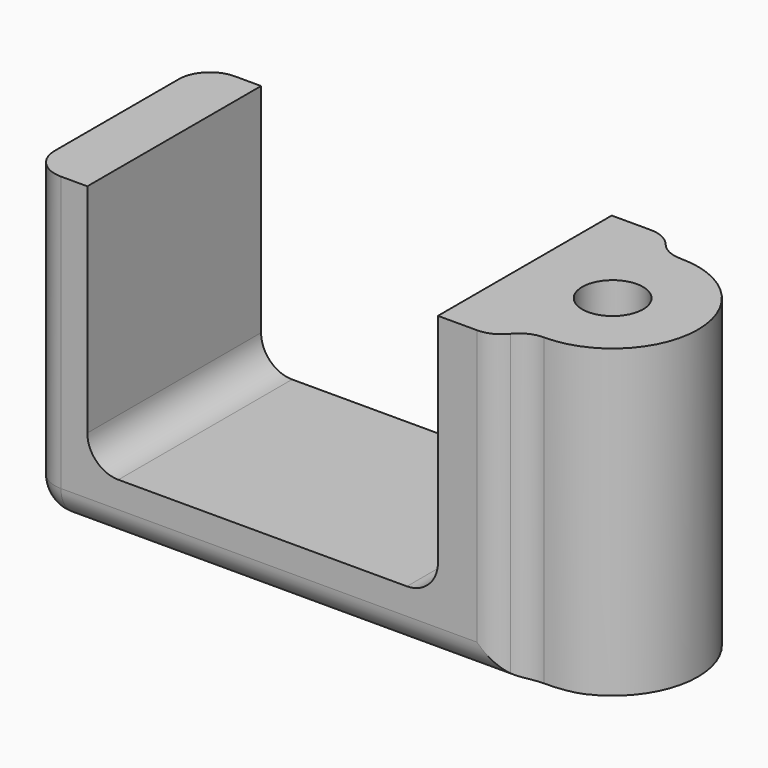
from build123d import *

# Parameters (mm, degrees)
F0_W         = 1.85
F0_H         = 7
F0_W_2       = 11.3
F1_DEPTH     = 1.85
F2_DEPTH     = 8
F3_T1_DEPTH  = 9.85
F3_T3_DEPTH  = 9.85
F3_T5_DEPTH  = 7
F3_T7_DEPTH  = 7
F3_T9_DEPTH  = 12
F4_T1_DEPTH  = 11.35
F4_T3_DEPTH  = 16.5
F4_T5_DEPTH  = 12.8150682373
F4_T8_ANGLE  = 90.0000000053
F4_T10_ANGLE = 90.0000000053


# Not quite as in the source:
# - a fillet or chamfer that OpenCascade refuses, or shapes differently, is made with other operations: its cross-section is extruded or revolved along the edge and cut away or added


with BuildPart() as f1:
    # F0 (on Top) → F1 (new body)
    with BuildSketch(Plane.XY):
        with Locations((-6.575, 0)):
            Rectangle(F0_W, F0_H)
        Rectangle(F0_W_2, F0_H)
        with BuildLine():
            Line((7.5, 0), (7.5, 2.5694551952))
            ThreePointArc((7.5, 2.5694551952), (5.73, 0), (7.5, -2.5694551952))
            Line((7.5, -2.5694551952), (7.5, 0))
        make_face()
        with BuildLine():
            Line((7.5, 2.5694551952), (7.5, 3.5))
            Line((7.5, 3.5), (5.65, 3.5))
            Line((5.65, 3.5), (5.65, -3.5))
            Line((5.65, -3.5), (7.5, -3.5))
            Line((7.5, -3.5), (7.5, -2.5694551952))
            ThreePointArc((7.5, -2.5694551952), (5.73, 0), (7.5, 2.5694551952))
        make_face()
        with BuildLine():
            ThreePointArc((11.23, 0), (10.0400480762, 2.2646743695), (7.5, 2.5694551952))
            Line((7.5, 2.5694551952), (7.5, 0))
            Line((7.5, 0), (7.5, -2.5694551952))
            ThreePointArc((7.5, -2.5694551952), (10.0400480762, -2.2646743695), (11.23, 0))
        make_face()
        with BuildLine():
            ThreePointArc((9.46, 0), (8.48, -0.98), (7.5, 0))
            ThreePointArc((7.5, 0), (8.48, 0.98), (9.46, 0))
        make_face(mode=Mode.SUBTRACT)
    extrude(amount=-F1_DEPTH)

    # F0 (on Top) → F2 (join)
    with BuildSketch(Plane.XY):
        with Locations((-6.575, 0)):
            Rectangle(F0_W, F0_H)
        with BuildLine():
            Line((7.5, 2.5694551952), (7.5, 3.5))
            Line((7.5, 3.5), (5.65, 3.5))
            Line((5.65, 3.5), (5.65, -3.5))
            Line((5.65, -3.5), (7.5, -3.5))
            Line((7.5, -3.5), (7.5, -2.5694551952))
            ThreePointArc((7.5, -2.5694551952), (5.73, 0), (7.5, 2.5694551952))
        make_face()
        with BuildLine():
            Line((7.5, 0), (7.5, 2.5694551952))
            ThreePointArc((7.5, 2.5694551952), (5.73, 0), (7.5, -2.5694551952))
            Line((7.5, -2.5694551952), (7.5, 0))
        make_face()
        with BuildLine():
            ThreePointArc((11.23, 0), (10.0400480762, 2.2646743695), (7.5, 2.5694551952))
            Line((7.5, 2.5694551952), (7.5, 0))
            Line((7.5, 0), (7.5, -2.5694551952))
            ThreePointArc((7.5, -2.5694551952), (10.0400480762, -2.2646743695), (11.23, 0))
        make_face()
        with BuildLine():
            ThreePointArc((9.46, 0), (8.48, -0.98), (7.5, 0))
            ThreePointArc((7.5, 0), (8.48, 0.98), (9.46, 0))
        make_face(mode=Mode.SUBTRACT)
    extrude(amount=F2_DEPTH)

    # F3: fillet of radius 1 on 5 edges, made by hand

    # F3_s2 → F3_t1 (join)
    with BuildSketch(Plane.XY.offset(-1.85)):
        with BuildLine():
            ThreePointArc((7.5, 3.5), (7.8571098794, 2.9584596209), (8.4713837652, 2.7499865019))
            ThreePointArc((8.4713837652, 2.7499865019), (7.9775177584, 2.7037033116), (7.5, 2.5694551952))
            Line((7.5, 2.5694551952), (7.5, 3.5))
        make_face()
    extrude(amount=F3_T1_DEPTH)

    # F3_s4 → F3_t3 (join)
    with BuildSketch(Plane.XY.offset(-1.85)):
        with BuildLine():
            ThreePointArc((7.5, -3.5), (7.8571098794, -2.9584596209), (8.4713837652, -2.7499865019))
            ThreePointArc((8.4713837652, -2.7499865019), (7.9775177584, -2.7037033116), (7.5, -2.5694551952))
            Line((7.5, -2.5694551952), (7.5, -3.5))
        make_face()
    extrude(amount=F3_T3_DEPTH)

    # F3_s6 → F3_t5 (join)
    with BuildSketch(Plane.XZ.offset(-3.5)):
        with BuildLine():
            ThreePointArc((5.65, 1), (5.3571067812, 0.2928932188), (4.65, 0))
            Line((4.65, 0), (5.65, 0))
            Line((5.65, 0), (5.65, 1))
        make_face()
    extrude(amount=F3_T5_DEPTH)

    # F3_s8 → F3_t7 (join)
    with BuildSketch(Plane.XZ.offset(-3.5)):
        with BuildLine():
            ThreePointArc((-4.65, 0), (-5.3571067812, 0.2928932188), (-5.65, 1))
            Line((-5.65, 1), (-5.65, 0))
            Line((-5.65, 0), (-4.65, 0))
        make_face()
    extrude(amount=F3_T7_DEPTH)

    # F3_s10 → F3_t9 (cut)
    with BuildSketch(Plane.XZ.offset(-6)):
        with BuildLine():
            ThreePointArc((-7.5, -0.85), (-7.2071067812, -1.5571067812), (-6.5, -1.85))
            Line((-6.5, -1.85), (-7.5, -1.85))
            Line((-7.5, -1.85), (-7.5, -0.85))
        make_face()
    extrude(amount=F3_T9_DEPTH, mode=Mode.SUBTRACT)

    # F4: fillet of radius 1 on 8 edges, made by hand

    # F4_s2 → F4_t1 (cut)
    with BuildSketch(Plane.XY.offset(-0.85)):
        with BuildLine():
            ThreePointArc((-7.5, 2.5), (-7.2071067812, 3.2071067812), (-6.5, 3.5))
            Line((-6.5, 3.5), (-7.5, 3.5))
            Line((-7.5, 3.5), (-7.5, 2.5))
        make_face()
        with BuildLine():
            ThreePointArc((-7.5, -2.5), (-7.2071067812, -3.2071067812), (-6.5, -3.5))
            Line((-6.5, -3.5), (-7.5, -3.5))
            Line((-7.5, -3.5), (-7.5, -2.5))
        make_face()
    extrude(amount=F4_T1_DEPTH, mode=Mode.SUBTRACT)

    # F4_s4 → F4_t3 (cut)
    with BuildSketch(Plane.YZ.offset(-6.5)):
        with BuildLine():
            ThreePointArc((3.5, -0.85), (3.2071067812, -1.5571067812), (2.5, -1.85))
            Line((2.5, -1.85), (3.5, -1.85))
            Line((3.5, -1.85), (3.5, -0.85))
        make_face()
        with BuildLine():
            ThreePointArc((-3.5, -0.85), (-3.2071067812, -1.5571067812), (-2.5, -1.85))
            Line((-2.5, -1.85), (-3.5, -1.85))
            Line((-3.5, -1.85), (-3.5, -0.85))
        make_face()
    extrude(amount=F4_T3_DEPTH, mode=Mode.SUBTRACT)

    # F4_s6 → F4_t5 (cut)
    with BuildSketch(Plane.XY.offset(-3.3325341187)):
        with BuildLine():
            ThreePointArc((6.9069863525, 3.5), (7.3400043679, 3.4013852663), (7.6876184707, 3.1249907968))
            ThreePointArc((7.6876184707, 3.1249907968), (7.5739320459, 3.3025507681), (7.5, 3.5))
            Line((7.5, 3.5), (6.9069863525, 3.5))
        make_face()
        with BuildLine():
            ThreePointArc((6.9069863525, -3.5), (7.3400043679, -3.4013852663), (7.6876184707, -3.1249907968))
            ThreePointArc((7.6876184707, -3.1249907968), (7.5739320459, -3.3025507681), (7.5, -3.5))
            Line((7.5, -3.5), (6.9069863525, -3.5))
        make_face()
    extrude(amount=F4_T5_DEPTH, mode=Mode.SUBTRACT)

    # F4_s7 → F4_t8 (revolve, cut)
    with BuildSketch(Plane.YZ.offset(-6.5)):
        with BuildLine():
            ThreePointArc((3.5, -0.85), (3.2071067812, -1.5571067812), (2.5, -1.85))
            Line((2.5, -1.85), (3.5, -1.85))
            Line((3.5, -1.85), (3.5, -0.85))
        make_face()
    revolve(axis=Axis((-6.5, 3.5, -0.85), (0, 1, 0)), revolution_arc=F4_T8_ANGLE, mode=Mode.SUBTRACT)

    # F4_s9 → F4_t10 (revolve, cut)
    with BuildSketch(Plane.YZ.offset(-6.5)):
        with BuildLine():
            ThreePointArc((-3.5, -0.85), (-3.2071067812, -1.5571067812), (-2.5, -1.85))
            Line((-2.5, -1.85), (-3.5, -1.85))
            Line((-3.5, -1.85), (-3.5, -0.85))
        make_face()
    revolve(axis=Axis((-6.5, -3.5, -0.85), (0, 1, 0)), revolution_arc=F4_T10_ANGLE, mode=Mode.SUBTRACT)


solid = f1.part
